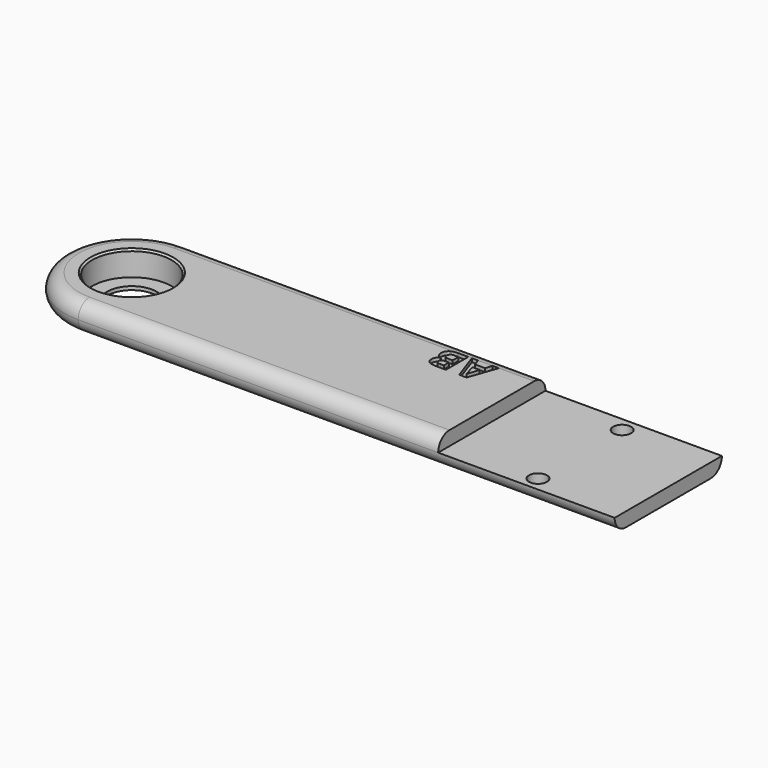
from build123d import *

# Parameters (mm, degrees)
F0_R          = 11.25
F1_DEPTH      = 8
F2_R          = 11.25
F2_R_2        = 7
F3_DEPTH      = 1
F5_ANGLE      = 90
F7_DEPTH      = 21
F8_R          = 3.99999
F10_D         = 5.08
F11_TEXT_SIZE = 11.1111111111
F12_DEPTH     = 1
F13_SIZE      = 0.5


# Not quite as in the source:
# - a fillet or chamfer is up to 0.001 mm smaller than in the source, because OpenCascade refuses the exact size
# - Text() gives the source's letters only with a copy of the font that has no kerning and outlines rounded to 1/6400 em; it was checked with that copy


with BuildPart() as f1:
    # F0 (on Top) → F1 (new body)
    with BuildSketch(Plane.XY):
        with BuildLine():
            Line((127, 19), (-127, 19))
            ThreePointArc((-127, 19), (-146, 0), (-127, -19))
            Line((-127, -19), (127, -19))
            ThreePointArc((127, -19), (146, 0), (127, 19))
        make_face()
        with Locations((-127, 0)):
            Circle(F0_R, mode=Mode.SUBTRACT)
        with Locations((127, 0)):
            Circle(F0_R, mode=Mode.SUBTRACT)
        with Locations((127, 0)):
            Circle(F0_R)
    extrude(amount=-F1_DEPTH)

    # F2 (on face) → F3 (join)
    with BuildSketch(Plane(origin=(0, 0, -8), x_dir=(1, 0, 0), z_dir=(0, 0, -1))):
        with Locations((-127, 0)):
            Circle(F2_R)
        with Locations((-127, 0)):
            Circle(F2_R_2, mode=Mode.SUBTRACT)
    extrude(amount=-F3_DEPTH)

    # F4 (on Front) → F5 (revolve)
    with BuildSketch(Plane.XZ):
        Polygon((131, -8), (129, -8), (129, -17.5), (131, -17.5), (131, -16), align=None)
        with BuildLine():
            Line((132.5, -16), (131, -16))
            Line((131, -16), (131, -17.5))
            Line((131, -17.5), (132.5, -17.5))
            ThreePointArc((132.5, -17.5), (132.8535533906, -17.3535533906), (133, -17))
            Line((133, -17), (133, -16.5))
            ThreePointArc((133, -16.5), (132.8535533906, -16.1464466094), (132.5, -16))
        make_face()
    revolve(axis=Axis((127, 0, -7), (0, 0, 1)), revolution_arc=F5_ANGLE)

    # F6 (on Front) → F7 (cut, symmetric)
    with BuildSketch(Plane.XZ):
        Polygon((-25, 0), (-25, -4), (25, -4), (25, -8), (152.5536179543, -37.6762710512), (152.5536179543, 13.4500768036), align=None)
    extrude(amount=F7_DEPTH, both=True, mode=Mode.SUBTRACT)

    # F8 (radius 4 in the source; OpenCascade refuses exactly that, so slightly less here)
    f8_edges = [f1.edges().sort_by_distance(p)[0] for p in [
        (-76, -19, 0),
        (-51, -19, -8),
    ]]
    fillet(f8_edges, radius=F8_R)

    # F10 (through all)
    with Locations(Plane.XY.offset(-4)):
        with Locations((0, 14.9), (0, -14.9)):
            Hole(F10_D / 2)

    # F11 (on face) → F12 (cut)
    with BuildSketch(Plane.XY):
        with Locations(Location((-35, 15), (0, 0, 180))):
            Text('AB', F11_TEXT_SIZE, font='Open Sans', font_style=FontStyle.BOLD, text_align=(TextAlign.LEFT, TextAlign.BOTTOM))
    extrude(amount=-F12_DEPTH, mode=Mode.SUBTRACT)

    # F13
    f13_edges = [f1.edges().sort_by_distance(p)[0] for p in [
        (-138.25, 0, 0),
    ]]
    chamfer(f13_edges, length=F13_SIZE)


solid = f1.part
